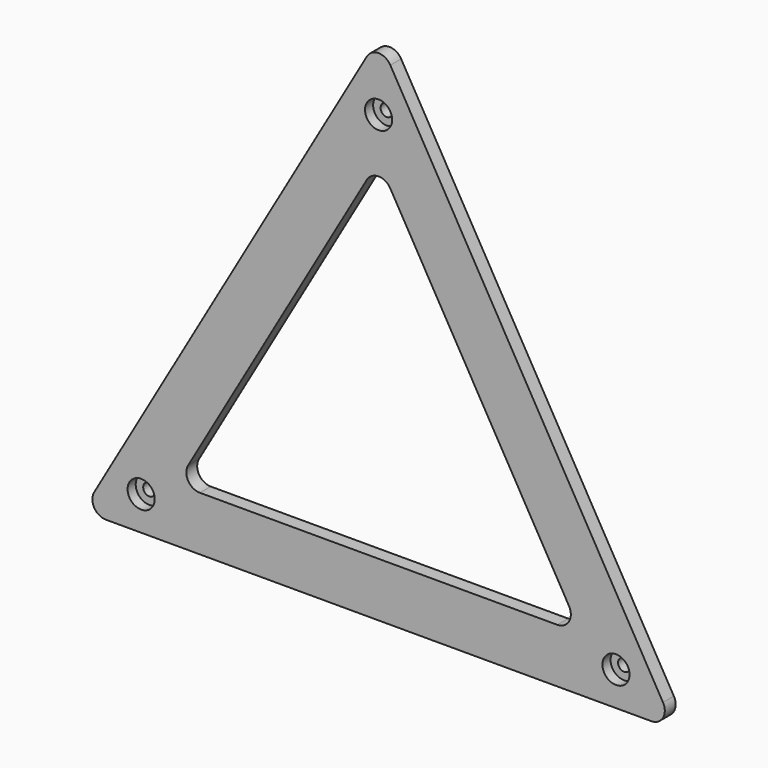
from build123d import *

# Parameters (mm, degrees)
F1_DEPTH       = 2
F2_R           = 2
F2_R_2         = 0.9
F3_DEPTH       = 2
F5_D           = 1.8
F5_CBORE_D     = 4
F5_CBORE_DEPTH = 1.5


# Not quite as in the source:
# - after a boolean that leaves OpenCascade's solid faulty, fix() repairs it


with BuildPart() as f1:
    # F0 (on Front) → F1 (new body)
    with BuildSketch(Plane.XZ):
        with BuildLine():
            ThreePointArc((1.7320509844, 47.5114831651), (1.769e-07, 48.5114831651), (-1.7320506307, 47.5114831651))
            Line((-1.7320506307, 47.5114831651), (-41.9318474004, -22.1166072941))
            ThreePointArc((-41.9318474004, -22.1166072941), (-41.9318474004, -24.1166072941), (-40.1997965929, -25.1166072941))
            Line((-40.1997965929, -25.1166072941), (40.1997969466, -25.1166072941))
            ThreePointArc((40.1997969466, -25.1166072941), (41.9318477542, -24.1166072941), (41.9318477542, -22.1166072941))
            Line((41.9318477542, -22.1166072941), (1.7320509844, 47.5114831651))
        make_face()
        with BuildLine():
            ThreePointArc((-1.7320506307, 31.5114831651), (1.769e-07, 32.5114831651), (1.7320509844, 31.5114831651))
            Line((1.7320509844, 31.5114831651), (28.0754412936, -14.1166072941))
            ThreePointArc((28.0754412936, -14.1166072941), (28.0754412936, -16.1166072941), (26.343390486, -17.1166072941))
            Line((26.343390486, -17.1166072941), (-26.3433901323, -17.1166072941))
            ThreePointArc((-26.3433901323, -17.1166072941), (-28.0754409399, -16.1166072941), (-28.0754409399, -14.1166072941))
            Line((-28.0754409399, -14.1166072941), (-1.7320506307, 31.5114831651))
        make_face(mode=Mode.SUBTRACT)
    extrude(amount=F1_DEPTH)

    # F2 (on face) → F3 (join)
    with BuildSketch(Plane(origin=(0, 0, 0), x_dir=(-1, 0, 0), z_dir=(0, 1, 0))):
        with Locations((-1.769e-07, 40.5114831651)):
            Circle(F2_R)
        with Locations((-1.769e-07, 40.5114831651)):
            Circle(F2_R_2, mode=Mode.SUBTRACT)
        with Locations((-35.0036445239, -20.1166072941)):
            Circle(F2_R)
        with Locations((-35.0036445239, -20.1166072941)):
            Circle(F2_R_2, mode=Mode.SUBTRACT)
        with Locations((35.0036441701, -20.1166072941)):
            Circle(F2_R)
        with Locations((35.0036441701, -20.1166072941)):
            Circle(F2_R_2, mode=Mode.SUBTRACT)
    extrude(amount=F3_DEPTH)

    # F5 (through all)
    with Locations(Plane.XZ.offset(2)):
        with Locations((1.769e-07, 40.5114831651), (-35.0036441701, -20.1166072941), (35.0036445239, -20.1166072941)):
            CounterBoreHole(F5_D / 2, F5_CBORE_D / 2, F5_CBORE_DEPTH)

    add(f1.part.fix(), mode=Mode.REPLACE)


solid = f1.part
